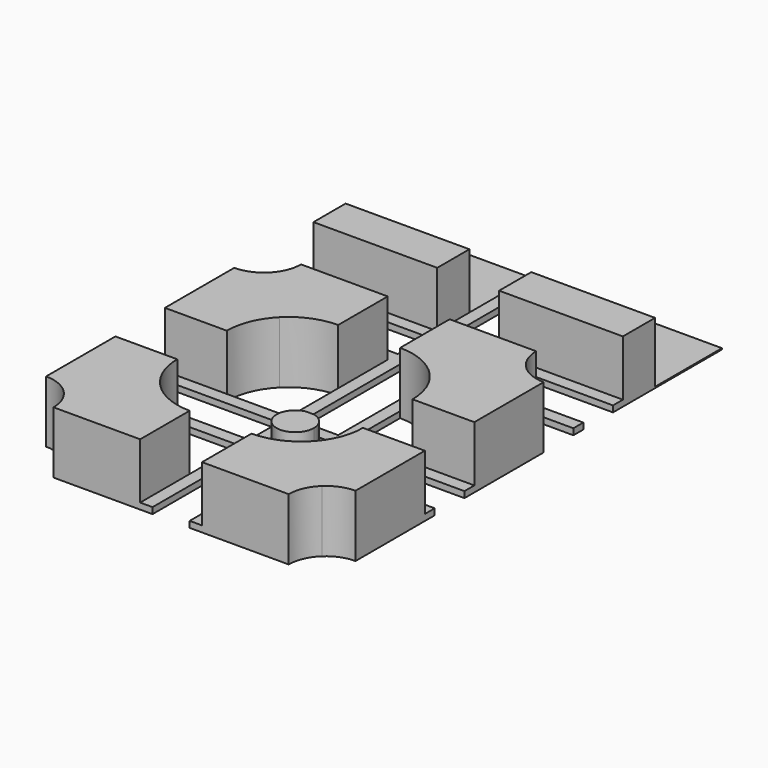
from build123d import *

# Parameters (mm, degrees)
F1_DEPTH = 5.08
F0_W     = 7.62
F0_H     = 7.62
F0_H_2   = 2.54
F0_W_2   = 2.54
F0_W_3   = 25.4
F2_DEPTH = 1.27
F0_H_3   = 8.2517393589
F3_DEPTH = 12.7
F0_H_4   = 17.1482606411
F4_DEPTH = 0.254


with BuildPart() as f1:
    # F0 (on Top) → F1 (new body)
    with BuildSketch(Plane.XY):
        with BuildLine():
            ThreePointArc((11.8236929674, -15.24), (9.6912048674, -16.5785939593), (8.8592705512, -18.954982938))
            ThreePointArc((8.8592705512, -18.954982938), (12.6692705296, -22.7649829811), (16.4792705512, -18.9549829811))
            ThreePointArc((16.4792705512, -18.9549829811), (15.6473362485, -16.5785939761), (13.514848135, -15.24))
            Line((13.514848135, -15.24), (11.8236929674, -15.24))
        make_face()
    extrude(amount=F1_DEPTH)


with BuildPart() as f2:
    # F0 (on Top) → F2 (new body)
    with BuildSketch(Plane.XY):
        Polygon((8.8592705512, 50.8), (6.3192705512, 50.8), (6.3192705512, 33.6517393589), (6.3192705512, 25.4), (8.8592705512, 25.4), align=None)
        Polygon((16.4792705512, 50.8), (16.4792705512, 25.4), (19.0192705512, 25.4), (19.0192705512, 33.6517393589), (19.0192705512, 50.8), align=None)
        with Locations((12.6692705512, 19.05)):
            Rectangle(F0_W, F0_H)
        with Locations((12.6692705512, 24.13)):
            Rectangle(F0_W, F0_H_2)
        with Locations((7.5892705512, 24.13)):
            Rectangle(F0_W_2, F0_H_2)
        with Locations((-6.3807294488, 24.13)):
            Rectangle(F0_W_3, F0_H_2)
        with Locations((7.5892705512, 19.05)):
            Rectangle(F0_W_2, F0_H)
        with Locations((17.7492705512, 19.05)):
            Rectangle(F0_W_2, F0_H)
        with Locations((31.7192705512, 24.13)):
            Rectangle(F0_W_3, F0_H_2)
        with Locations((17.7492705512, 24.13)):
            Rectangle(F0_W_2, F0_H_2)
        Polygon((44.4192705512, 15.24), (19.0192705512, 15.24), (19.0192705512, 12.7), (36.7992705512, 12.7), (44.4192705512, 12.7), align=None)
        with Locations((17.7492705512, 13.97)):
            Rectangle(F0_W_2, F0_H_2)
        with Locations((7.5892705512, 13.97)):
            Rectangle(F0_W_2, F0_H_2)
        Polygon((6.3192705512, 12.7), (6.3192705512, 15.24), (-19.0807294488, 15.24), (-19.0807294488, 12.7), (-11.4607294488, 12.7), align=None)
        with Locations((12.6692705512, 13.97)):
            Rectangle(F0_W, F0_H_2)
        Polygon((8.8592705512, 12.7), (6.3192705512, 12.7), (6.3192705512, 0), (6.3192705512, -12.7), (8.8592705512, -12.7), align=None)
        Polygon((19.0192705512, 12.7), (16.4792705512, 12.7), (16.4792705512, -12.7), (19.0192705512, -12.7), (19.0192705512, 0), align=None)
        Polygon((6.3192705512, -15.24), (6.3192705512, -12.7), (-6.3807294488, -12.7), (-19.0807294488, -12.7), (-19.0807294488, -15.24), align=None)
        with Locations((7.5892705512, -13.97)):
            Rectangle(F0_W_2, F0_H_2)
        with BuildLine():
            Line((16.4792705512, -12.7), (8.8592705512, -12.7))
            Line((8.8592705512, -12.7), (8.8592705512, -15.24))
            Line((8.8592705512, -15.24), (11.8236929674, -15.24))
            ThreePointArc((11.8236929674, -15.24), (12.6692705512, -15.1449829811), (13.514848135, -15.24))
            Line((13.514848135, -15.24), (16.4792705512, -15.24))
            Line((16.4792705512, -15.24), (16.4792705512, -12.7))
        make_face()
        with Locations((17.7492705512, -13.97)):
            Rectangle(F0_W_2, F0_H_2)
        Polygon((31.7192705512, -12.7), (19.0192705512, -12.7), (19.0192705512, -15.24), (44.4192705512, -15.24), (44.4192705512, -12.7), align=None)
        Polygon((19.0192705512, -15.24), (16.4792705512, -15.24), (16.4792705512, -18.9549829811), (16.4792705512, -22.86), (19.0192705512, -22.86), align=None)
        Polygon((8.8592705512, -18.954982938), (8.8592705512, -15.24), (6.3192705512, -15.24), (6.3192705512, -22.86), (8.8592705512, -22.86), align=None)
        with Locations((12.6692705512, -24.13)):
            Rectangle(F0_W, F0_H_2)
        with Locations((7.5892705512, -24.13)):
            Rectangle(F0_W_2, F0_H_2)
        Polygon((6.3192705512, -25.4), (6.3192705512, -22.86), (-19.0807294488, -22.86), (-19.0807294488, -25.4), (-6.3807294488, -25.4), align=None)
        Polygon((44.4192705512, -22.86), (19.0192705512, -22.86), (19.0192705512, -25.4), (31.7192705512, -25.4), (44.4192705512, -25.4), align=None)
        with Locations((17.7492705512, -24.13)):
            Rectangle(F0_W_2, F0_H_2)
        Polygon((19.0192705512, -25.4), (16.4792705512, -25.4), (16.4792705512, -50.8), (19.0192705512, -50.8), (19.0192705512, -38.1), align=None)
        Polygon((8.8592705512, -25.4), (6.3192705512, -25.4), (6.3192705512, -38.1), (6.3192705512, -50.8), (8.8592705512, -50.8), align=None)
    extrude(amount=F2_DEPTH)

    # F0 (on Top) → F3 (join)
    with BuildSketch(Plane.XY):
        with Locations((-6.3807294488, 29.5258696795)):
            Rectangle(F0_W_3, F0_H_3)
        with Locations((31.7192705512, 29.5258696795)):
            Rectangle(F0_W_3, F0_H_3)
        with BuildLine():
            Line((6.3192705512, 0), (6.3192705512, 12.7))
            Line((6.3192705512, 12.7), (-11.4607294488, 12.7))
            ThreePointArc((-11.4607294488, 12.7), (-12.0854948202, 9.6782302386), (-13.8573416512, 7.151971529))
            ThreePointArc((-13.8573416512, 7.151971529), (-16.2710654964, 5.6169082687), (-19.0807294488, 5.08))
            Line((-19.0807294488, 5.08), (-19.0807294488, -12.7))
            Line((-19.0807294488, -12.7), (-6.3807294488, -12.7))
            ThreePointArc((-6.3807294488, -12.7), (-5.4233122083, -7.8624644563), (-2.6954144666, -3.7543052797))
            ThreePointArc((-2.6954144666, -3.7543052797), (1.4366648405, -0.9760859149), (6.3192705512, 0))
        make_face()
        with BuildLine():
            Line((36.7992705512, 12.7), (19.0192705512, 12.7))
            Line((19.0192705512, 12.7), (19.0192705512, 0))
            ThreePointArc((19.0192705512, 0), (24.108011302, -1.0640764195), (28.34402622, -4.0779972329))
            ThreePointArc((28.34402622, -4.0779972329), (30.8453941129, -8.0704426234), (31.7192705512, -12.7))
            Line((31.7192705512, -12.7), (44.4192705512, -12.7))
            Line((44.4192705512, -12.7), (44.4192705512, 5.08))
            ThreePointArc((44.4192705512, 5.08), (41.3795616585, 5.7125419609), (38.8445098324, 7.505152271))
            ThreePointArc((38.8445098324, 7.505152271), (37.3289928177, 9.9085198082), (36.7992705512, 12.7))
        make_face()
        with BuildLine():
            Line((44.4192705512, -25.4), (31.7192705512, -25.4))
            ThreePointArc((31.7192705512, -25.4), (30.9285782234, -29.8111665996), (28.6549570442, -33.6730614532))
            ThreePointArc((28.6549570442, -33.6730614532), (24.3212569499, -36.9403180298), (19.0192705512, -38.1))
            Line((19.0192705512, -38.1), (19.0192705512, -50.8))
            Line((19.0192705512, -50.8), (36.7992705512, -50.8))
            ThreePointArc((36.7992705512, -50.8), (37.4241240621, -47.7780262087), (39.1962064031, -45.2516668355))
            ThreePointArc((39.1962064031, -45.2516668355), (41.6098131938, -43.7168263217), (44.4192705512, -43.18))
            Line((44.4192705512, -43.18), (44.4192705512, -25.4))
        make_face()
        with BuildLine():
            ThreePointArc((-1.7277739655, -35.2252264374), (-5.1586967201, -30.8356478288), (-6.3807294488, -25.4))
            Line((-6.3807294488, -25.4), (-19.0807294488, -25.4))
            Line((-19.0807294488, -25.4), (-19.0807294488, -43.18))
            ThreePointArc((-19.0807294488, -43.18), (-16.155204139, -43.7639711725), (-13.6780836704, -45.4263775167))
            ThreePointArc((-13.6780836704, -45.4263775167), (-12.0368469671, -47.8934350886), (-11.4607294488, -50.8))
            Line((-11.4607294488, -50.8), (6.3192705512, -50.8))
            Line((6.3192705512, -50.8), (6.3192705512, -38.1))
            ThreePointArc((6.3192705512, -38.1), (2.0467054993, -37.3597319317), (-1.7277739655, -35.2252264374))
        make_face()
    extrude(amount=F3_DEPTH)

    # F0 (on Top) → F4 (join)
    with BuildSketch(Plane.XY):
        with Locations((-6.3807294488, 42.2258696795)):
            Rectangle(F0_W_3, F0_H_4)
        with Locations((31.7192705512, 42.2258696795)):
            Rectangle(F0_W_3, F0_H_4)
    extrude(amount=F4_DEPTH)


solid = Compound([f1.part, f2.part])
